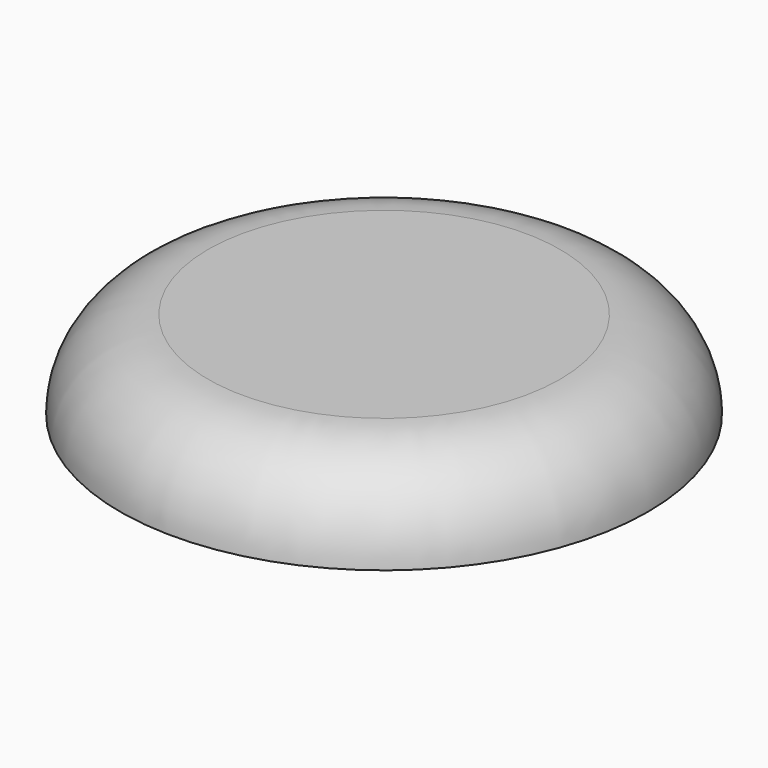
from build123d import *

# Parameters (mm, degrees)
F0_R     = 15
F1_DEPTH = 5
F2_R     = 4.99999


# Not quite as in the source:
# - a fillet or chamfer is up to 0.001 mm smaller than in the source, because OpenCascade refuses the exact size


with BuildPart() as f1:
    # F0 (on Top) → F1 (new body)
    with BuildSketch(Plane.XY):
        with Locations((-40.5482724309, 37.26311028)):
            Circle(F0_R)
    extrude(amount=F1_DEPTH)

    # F2 (radius 5 in the source; OpenCascade refuses exactly that, so slightly less here)
    f2_edges = [f1.edges().sort_by_distance(p)[0] for p in [
        (-55.548272, 37.26311, 5),
    ]]
    fillet(f2_edges, radius=F2_R)


solid = f1.part
